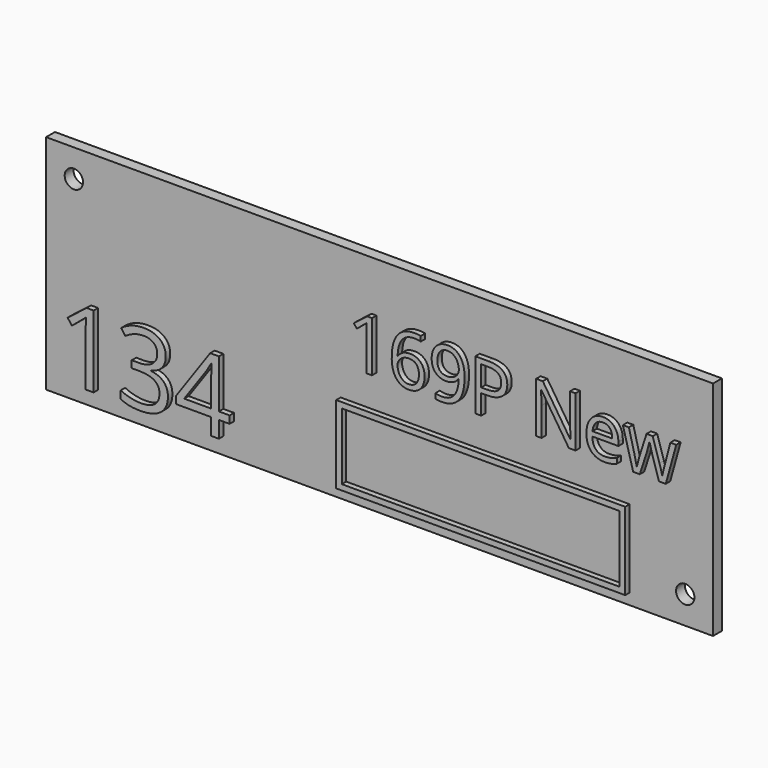
from build123d import *

# Parameters (mm, degrees)
F0_W         = 120
F0_H         = 40
F1_DEPTH     = 2
F3_D         = 3.3
F4_TEXT_SIZE = 12.7013528264
F5_DEPTH     = 1
F6_TEXT_SIZE = 18.1818181818
F7_DEPTH     = 1
F8_W         = 52
F8_H         = 14
F8_W_2       = 49.99999962
F8_H_2       = 11.99999962
F9_DEPTH     = 1


# Not quite as in the source:
# - Text() gives the source's letters only with a copy of the font that has no kerning and outlines rounded to 1/6400 em; it was checked with that copy


with BuildPart() as f1:
    # F0 (on Front) → F1 (new body)
    with BuildSketch(Plane.XZ):
        Rectangle(F0_W, F0_H)
    extrude(amount=F1_DEPTH)

    # F3 (through all)
    with Locations(Plane.XZ.offset(2)):
        with Locations((-55, 15), (55, -15)):
            Hole(F3_D / 2)

    # F4 (on face) → F5 (join)
    with BuildSketch(Plane.XZ.offset(2)):
        with Locations((-5, 2)):
            Text('169P New', F4_TEXT_SIZE, font='Open Sans', text_align=(TextAlign.LEFT, TextAlign.BOTTOM))
    extrude(amount=F5_DEPTH)

    # F6 (on face) → F7 (join)
    with BuildSketch(Plane.XZ.offset(2)):
        with Locations((-57, -17)):
            Text('134', F6_TEXT_SIZE, font='Open Sans', text_align=(TextAlign.LEFT, TextAlign.BOTTOM))
    extrude(amount=F7_DEPTH)

    # F8 (on face) → F9 (join)
    with BuildSketch(Plane.XZ.offset(2)):
        with Locations((19, -11)):
            Rectangle(F8_W, F8_H)
        with Locations((19, -11)):
            Rectangle(F8_W_2, F8_H_2, mode=Mode.SUBTRACT)
    extrude(amount=F9_DEPTH)


solid = f1.part
